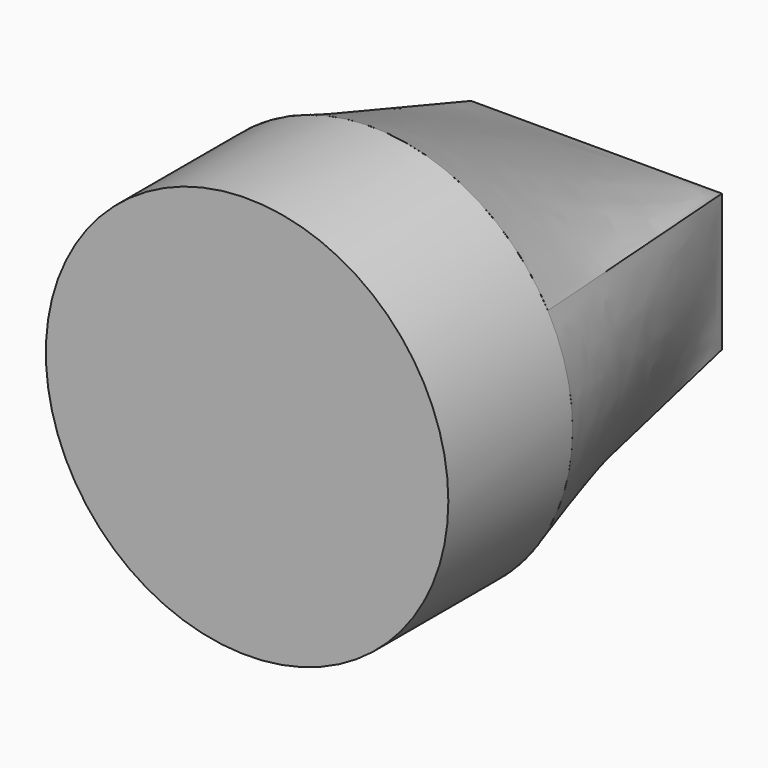
from build123d import *

# Parameters (mm, degrees)
F2_R     = 35.7602314712
F3_DEPTH = 27.59926
F0_W     = 44.5784255862
F0_H     = 24.4192462415


# Not quite as in the source:
# - the arcs of a loft's sections are written as splines that run evenly, so that the points pair up as in the source's solid


with BuildPart() as f3:
    # F2 (on offset) → F3 (new body)
    with BuildSketch(Plane.XZ.offset(50)):
        Circle(F2_R)
    extrude(amount=F3_DEPTH)


with BuildPart() as f4:
    # F3_face (on face) → F4 section 0
    with BuildSketch(Plane(origin=(0, -50, 0), x_dir=(1, 0, 0), z_dir=(0, 1, 0))):
        with BuildLine():
            add(Edge.make_bspline(
                [(31.3630160959, -17.1800866192), (32.4874501357, -15.1273820159), (33.4096876137, -12.9639838215), (34.8144187197, -8.4987265037), (35.2968776128, -6.1969777925), (35.8034887164, -1.5434696982), (35.8276283999, 0.8081746177), (35.4166507206, 5.4711017822), (34.9815435199, 7.7822693307), (33.6687706994, 12.2754218894), (32.7911375404, 14.4572957976), (30.627018702, 18.6080044175), (29.3405865347, 20.5767364947), (26.4082875517, 24.2254917713), (24.7624932428, 25.905424748), (21.1747007207, 28.9120070622), (19.2327912226, 30.2385820561), (17.1800866192, 31.3630160959)],
                knots=[0, 0, 0, 0, 0.125, 0.125, 0.25, 0.25, 0.375, 0.375, 0.5, 0.5, 0.625, 0.625, 0.75, 0.75, 0.875, 0.875, 1, 1, 1, 1], degree=3))
            add(Edge.make_bspline(
                [(17.1800866192, 31.3630160959), (15.1273820159, 32.4874501357), (12.9639838215, 33.4096876137), (8.4987265037, 34.8144187197), (6.1969777925, 35.2968776128), (1.5434696982, 35.8034887164), (-0.8081746177, 35.8276283999), (-5.4711017822, 35.4166507206), (-7.7822693307, 34.9815435199), (-12.2754218894, 33.6687706994), (-14.4572957976, 32.7911375404), (-18.6080044175, 30.627018702), (-20.5767364947, 29.3405865347), (-24.2254917713, 26.4082875517), (-25.905424748, 24.7624932428), (-28.9120070622, 21.1747007207), (-30.2385820561, 19.2327912226), (-31.3630160959, 17.1800866192)],
                knots=[0, 0, 0, 0, 0.125, 0.125, 0.25, 0.25, 0.375, 0.375, 0.5, 0.5, 0.625, 0.625, 0.75, 0.75, 0.875, 0.875, 1, 1, 1, 1], degree=3))
            add(Edge.make_bspline(
                [(-31.3630160959, 17.1800866192), (-32.4874501357, 15.1273820159), (-33.4096876137, 12.9639838215), (-34.8144187197, 8.4987265037), (-35.2968776128, 6.1969777925), (-35.8034887164, 1.5434696982), (-35.8276283999, -0.8081746177), (-35.4166507206, -5.4711017822), (-34.9815435199, -7.7822693307), (-33.6687706994, -12.2754218894), (-32.7911375404, -14.4572957976), (-30.627018702, -18.6080044175), (-29.3405865347, -20.5767364947), (-26.4082875517, -24.2254917713), (-24.7624932428, -25.905424748), (-21.1747007207, -28.9120070622), (-19.2327912226, -30.2385820561), (-17.1800866192, -31.3630160959)],
                knots=[0, 0, 0, 0, 0.125, 0.125, 0.25, 0.25, 0.375, 0.375, 0.5, 0.5, 0.625, 0.625, 0.75, 0.75, 0.875, 0.875, 1, 1, 1, 1], degree=3))
            add(Edge.make_bspline(
                [(-17.1800866192, -31.3630160959), (-15.1273820159, -32.4874501357), (-12.9639838215, -33.4096876137), (-8.4987265037, -34.8144187197), (-6.1969777925, -35.2968776128), (-1.5434696982, -35.8034887164), (0.8081746177, -35.8276283999), (5.4711017822, -35.4166507206), (7.7822693307, -34.9815435199), (12.2754218894, -33.6687706994), (14.4572957976, -32.7911375404), (18.6080044175, -30.627018702), (20.5767364947, -29.3405865347), (24.2254917713, -26.4082875517), (25.905424748, -24.7624932428), (28.9120070622, -21.1747007207), (30.2385820561, -19.2327912226), (31.3630160959, -17.1800866192)],
                knots=[0, 0, 0, 0, 0.125, 0.125, 0.25, 0.25, 0.375, 0.375, 0.5, 0.5, 0.625, 0.625, 0.75, 0.75, 0.875, 0.875, 1, 1, 1, 1], degree=3))
        make_face()
    # F0 (on Front) → F4 section 1
    with BuildSketch(Plane.XZ):
        Rectangle(F0_W, F0_H)
    loft(ruled=True)


solid = Compound([f3.part, f4.part])
